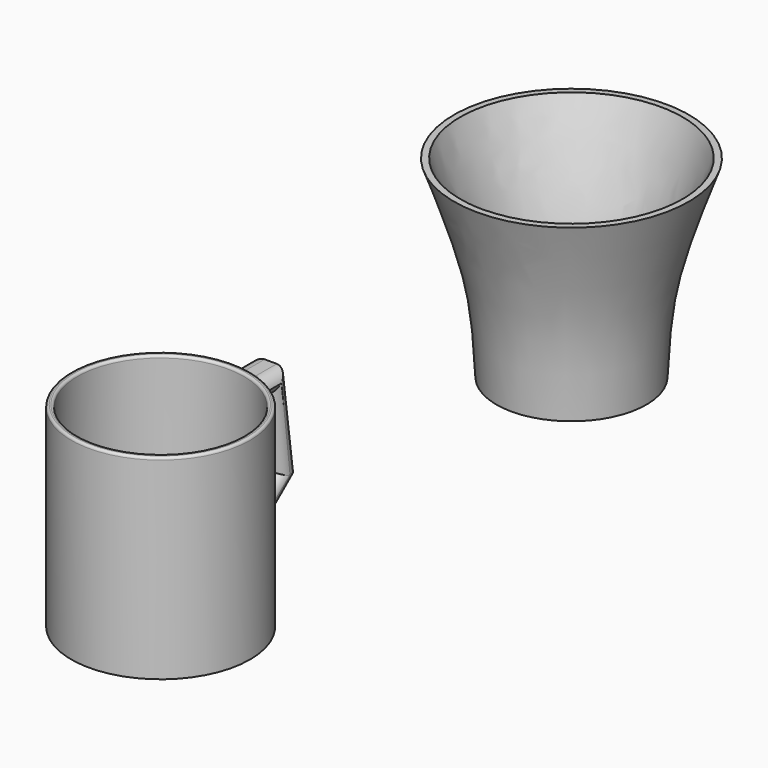
from build123d import *

# Parameters (mm, degrees)
F0_R          = 36.9971059263
F1_DEPTH      = 80.772
F2_T          = -2.54
F3_R          = 1
F5_DEPTH      = 7.5
F6_T1_DEPTH   = 65.9582815791
F6_T6_DEPTH   = 45.598795265
F6_S7_R       = 36.9971059263
F6_T8_DEPTH   = 25
F6_T12_DEPTH  = 57.9884008933
F6_S13_R      = 36.9971059263
F6_T14_DEPTH  = 33
F6_T18_DEPTH  = 44.3714568285
F6_S19_R      = 36.9971059263
F6_T20_DEPTH  = 26
F6_T25_DEPTH  = 54.3686230344
F6_T31_DEPTH  = 38.2201202214
F6_S32_R      = 36.9971059263
F6_T33_DEPTH  = 21
F6_T38_DEPTH  = 45.598795265
F6_S39_R      = 36.9971059263
F6_T40_DEPTH  = 25
F6_T44_DEPTH  = 38.2201202214
F6_S45_R      = 36.9971059263
F6_T46_DEPTH  = 21
F6_T51_DEPTH  = 54.3686230344
F6_T57_DEPTH  = 44.3714568285
F6_S58_R      = 36.9971059263
F6_T59_DEPTH  = 26
F6_T64_DEPTH  = 57.9884008933
F6_S65_R      = 36.9971059263
F6_T66_DEPTH  = 33
F6_T71_DEPTH  = 44.3714568285
F6_T76_DEPTH  = 54.3686230344
F6_T84_DEPTH  = 25.7201202214
F6_T89_DEPTH  = 54.3686230344
F6_T97_DEPTH  = 25.7201202214
F6_T102_DEPTH = 54.3686230344
F6_T110_DEPTH = 44.3714568285
F6_T115_DEPTH = 54.3686230344
F9_T          = -2.5


# Not quite as in the source:
# - a fillet or chamfer that OpenCascade refuses, or shapes differently, is made with other operations: its cross-section is extruded or revolved along the edge and cut away or added


with BuildPart() as f1:
    # F0 (on Top) → F1 (new body)
    with BuildSketch(Plane.XY):
        Circle(F0_R)
    extrude(amount=F1_DEPTH)

    # F2
    f2_openings = [f1.faces().sort_by_distance(p)[0] for p in [
        (0, 0, 80.772),
    ]]
    offset(amount=F2_T, openings=f2_openings)

    # F3
    f3_edges = [f1.edges().sort_by_distance(p)[0] for p in [
        (-34.457106, 0, 80.772),
        (-36.997106, 0, 80.772),
    ]]
    fillet(f3_edges, radius=F3_R)

    # F4 (on Right) → F5 (join, symmetric)
    with BuildSketch(Plane.YZ):
        Polygon((56.8772740662, 73.2908397913), (36.2784788013, 73.2908397913), (36.2784788013, 65.2972832322), (49.4985990226, 65.2972832322), (52.5730475783, 36.0900275409), (36.8933677673, 24.7145723552), (36.8933677673, 11.8018947542), (62.411274761, 32.7081382275), align=None)
    extrude(amount=F5_DEPTH, both=True)

    # F6: fillet of radius 5 on 12 edges, made by hand

    # F6_s2 → F6_t1 (cut)
    with BuildSketch(Plane(origin=(0, -1.5505079286, 11.3703998263), x_dir=(1, 0, 0), z_dir=(0, -0.1351131073, 0.9908301813))):
        with BuildLine():
            ThreePointArc((7.5, 61.2582728789), (6.0355339059, 64.7938067849), (2.5, 66.2582728789))
            Line((2.5, 66.2582728789), (7.5, 66.2582728789))
            Line((7.5, 66.2582728789), (7.5, 61.2582728789))
        make_face()
        with BuildLine():
            ThreePointArc((-7.5, 61.2582728789), (-6.0355339059, 64.7938067849), (-2.5, 66.2582728789))
            Line((-2.5, 66.2582728789), (-7.5, 66.2582728789))
            Line((-7.5, 66.2582728789), (-7.5, 61.2582728789))
        make_face()
    extrude(amount=F6_T1_DEPTH, mode=Mode.SUBTRACT)


with BuildPart() as f6_tool4:
    # F6_s5 → F6_t6 (new body)
    with BuildSketch(Plane.XZ.offset(-69.3772740662)):
        with BuildLine():
            ThreePointArc((2.5, 73.2908397913), (6.0355339059, 71.8263736972), (7.5, 68.2908397913))
            Line((7.5, 68.2908397913), (7.5, 73.2908397913))
            Line((7.5, 73.2908397913), (2.5, 73.2908397913))
        make_face()
    extrude(amount=F6_T6_DEPTH)

    # F6_s7 → F6_t8 (cut, symmetric)
    with BuildSketch(Plane.XY.offset(70.8)):
        Circle(F6_S7_R)
    extrude(amount=F6_T8_DEPTH, both=True, mode=Mode.SUBTRACT)


with BuildPart() as f1_1:
    add(f1.part)

    # F6_t3: cut F6_tool4
    add(f6_tool4.part, mode=Mode.SUBTRACT)


with BuildPart() as f6_tool10:
    # F6_s11 → F6_t12 (new body)
    with BuildSketch(Plane(origin=(0, 18.192122961, 14.9043944715), x_dir=(1, 0, 0), z_dir=(0, 0.7735417996, 0.6337452834))):
        with BuildLine():
            ThreePointArc((2.5, 14.2517389045), (6.0355339059, 12.7872728104), (7.5, 9.2517389045))
            Line((7.5, 9.2517389045), (7.5, 14.2517389045))
            Line((7.5, 14.2517389045), (2.5, 14.2517389045))
        make_face()
    extrude(amount=F6_T12_DEPTH)

    # F6_s13 → F6_t14 (cut, symmetric)
    with BuildSketch(Plane.XY.offset(24.2)):
        Circle(F6_S13_R)
    extrude(amount=F6_T14_DEPTH, both=True, mode=Mode.SUBTRACT)


with BuildPart() as f1_2:
    add(f1_1.part)

    # F6_t9: cut F6_tool10
    add(f6_tool10.part, mode=Mode.SUBTRACT)


with BuildPart() as f6_tool16:
    # F6_s17 → F6_t18 (new body)
    with BuildSketch(Plane(origin=(0, 61.7158510594, 44.7742496301), x_dir=(1, 0, 0), z_dir=(0, -0.8094218184, -0.587227656))):
        with BuildLine():
            ThreePointArc((2.5, -1.6602917777), (6.0355339059, -3.1247578718), (7.5, -6.6602917777))
            Line((7.5, -6.6602917777), (7.5, -1.6602917777))
            Line((7.5, -1.6602917777), (2.5, -1.6602917777))
        make_face()
    extrude(amount=F6_T18_DEPTH)

    # F6_s19 → F6_t20 (cut, symmetric)
    with BuildSketch(Plane.XY.offset(28.4)):
        Circle(F6_S19_R)
    extrude(amount=F6_T20_DEPTH, both=True, mode=Mode.SUBTRACT)

    split(bisect_by=Plane(origin=(0, 55.754223012, 5.868866703), x_dir=(1, 0, 0), z_dir=(0, -0.9945054508, -0.1046848043)), keep=Keep.TOP)


with BuildPart() as f1_3:
    add(f1_2.part)

    # F6_t15: cut F6_tool16
    add(f6_tool16.part, mode=Mode.SUBTRACT)


with BuildPart() as f6_tool23:
    # F6_s24 → F6_t25 (new body)
    with BuildSketch(Plane(origin=(0, -7.5641840435, 71.8597346646), x_dir=(1, 0, 0), z_dir=(0, 0.1046848043, -0.9945054508))):
        with BuildLine():
            ThreePointArc((7.5, -61.062259855), (6.0355339059, -57.5267259491), (2.5, -56.062259855))
            Line((2.5, -56.062259855), (7.5, -56.062259855))
            Line((7.5, -56.062259855), (7.5, -61.062259855))
        make_face()
    extrude(amount=F6_T25_DEPTH)

    split(bisect_by=Plane.XY.offset(65.2972832322), keep=Keep.BOTTOM)

    split(bisect_by=Plane(origin=(0, 0.9749692488, -1.3438763898), x_dir=(1, 0, 0), z_dir=(0, -0.587227656, 0.8094218184)), keep=Keep.TOP)


with BuildPart() as f1_4:
    add(f1_3.part)

    # F6_t22: cut F6_tool23
    add(f6_tool23.part, mode=Mode.SUBTRACT)


with BuildPart() as f6_tool29:
    # F6_s30 → F6_t31 (new body)
    with BuildSketch(Plane.XZ.offset(-23.7784788013)):
        with BuildLine():
            ThreePointArc((2.5, 65.2972832322), (6.0355339059, 66.7617493263), (7.5, 70.2972832322))
            Line((7.5, 70.2972832322), (7.5, 65.2972832322))
            Line((7.5, 65.2972832322), (2.5, 65.2972832322))
        make_face()
    extrude(amount=-F6_T31_DEPTH)

    # F6_s32 → F6_t33 (cut, symmetric)
    with BuildSketch(Plane.XY.offset(67.8)):
        Circle(F6_S32_R)
    extrude(amount=F6_T33_DEPTH, both=True, mode=Mode.SUBTRACT)

    split(bisect_by=Plane(origin=(0, 55.754223012, 5.868866703), x_dir=(1, 0, 0), z_dir=(0, -0.9945054508, -0.1046848043)), keep=Keep.TOP)


with BuildPart() as f1_5:
    add(f1_4.part)

    # F6_t28: cut F6_tool29
    add(f6_tool29.part, mode=Mode.SUBTRACT)


with BuildPart() as f6_tool36:
    # F6_s37 → F6_t38 (new body)
    with BuildSketch(Plane.XZ.offset(-69.3772740662)):
        with BuildLine():
            ThreePointArc((-2.5, 73.2908397913), (-6.0355339059, 71.8263736972), (-7.5, 68.2908397913))
            Line((-7.5, 68.2908397913), (-7.5, 73.2908397913))
            Line((-7.5, 73.2908397913), (-2.5, 73.2908397913))
        make_face()
    extrude(amount=F6_T38_DEPTH)

    # F6_s39 → F6_t40 (cut, symmetric)
    with BuildSketch(Plane.XY.offset(70.8)):
        Circle(F6_S39_R)
    extrude(amount=F6_T40_DEPTH, both=True, mode=Mode.SUBTRACT)


with BuildPart() as f1_6:
    add(f1_5.part)

    # F6_t35: cut F6_tool36
    add(f6_tool36.part, mode=Mode.SUBTRACT)


with BuildPart() as f6_tool42:
    # F6_s43 → F6_t44 (new body)
    with BuildSketch(Plane.XZ.offset(-23.7784788013)):
        with BuildLine():
            ThreePointArc((-2.5, 65.2972832322), (-6.0355339059, 66.7617493263), (-7.5, 70.2972832322))
            Line((-7.5, 70.2972832322), (-7.5, 65.2972832322))
            Line((-7.5, 65.2972832322), (-2.5, 65.2972832322))
        make_face()
    extrude(amount=-F6_T44_DEPTH)

    # F6_s45 → F6_t46 (cut, symmetric)
    with BuildSketch(Plane.XY.offset(67.8)):
        Circle(F6_S45_R)
    extrude(amount=F6_T46_DEPTH, both=True, mode=Mode.SUBTRACT)

    split(bisect_by=Plane(origin=(0, 55.754223012, 5.868866703), x_dir=(1, 0, 0), z_dir=(0, -0.9945054508, -0.1046848043)), keep=Keep.TOP)


with BuildPart() as f1_7:
    add(f1_6.part)

    # F6_t41: cut F6_tool42
    add(f6_tool42.part, mode=Mode.SUBTRACT)


with BuildPart() as f6_tool49:
    # F6_s50 → F6_t51 (new body)
    with BuildSketch(Plane(origin=(0, -7.5641840435, 71.8597346646), x_dir=(1, 0, 0), z_dir=(0, 0.1046848043, -0.9945054508))):
        with BuildLine():
            ThreePointArc((-2.5, -56.062259855), (-6.0355339059, -57.5267259491), (-7.5, -61.062259855))
            Line((-7.5, -61.062259855), (-7.5, -56.062259855))
            Line((-7.5, -56.062259855), (-2.5, -56.062259855))
        make_face()
    extrude(amount=F6_T51_DEPTH)

    split(bisect_by=Plane.XY.offset(65.2972832322), keep=Keep.BOTTOM)

    split(bisect_by=Plane(origin=(0, 0.9749692488, -1.3438763898), x_dir=(1, 0, 0), z_dir=(0, -0.587227656, 0.8094218184)), keep=Keep.TOP)


with BuildPart() as f1_8:
    add(f1_7.part)

    # F6_t48: cut F6_tool49
    add(f6_tool49.part, mode=Mode.SUBTRACT)


with BuildPart() as f6_tool55:
    # F6_s56 → F6_t57 (new body)
    with BuildSketch(Plane(origin=(0, 61.7158510594, 44.7742496301), x_dir=(1, 0, 0), z_dir=(0, -0.8094218184, -0.587227656))):
        with BuildLine():
            ThreePointArc((-2.5, -1.6602917777), (-6.0355339059, -3.1247578718), (-7.5, -6.6602917777))
            Line((-7.5, -6.6602917777), (-7.5, -1.6602917777))
            Line((-7.5, -1.6602917777), (-2.5, -1.6602917777))
        make_face()
    extrude(amount=F6_T57_DEPTH)

    # F6_s58 → F6_t59 (cut, symmetric)
    with BuildSketch(Plane.XY.offset(28.4)):
        Circle(F6_S58_R)
    extrude(amount=F6_T59_DEPTH, both=True, mode=Mode.SUBTRACT)

    split(bisect_by=Plane(origin=(0, 55.754223012, 5.868866703), x_dir=(1, 0, 0), z_dir=(0, -0.9945054508, -0.1046848043)), keep=Keep.TOP)


with BuildPart() as f1_9:
    add(f1_8.part)

    # F6_t54: cut F6_tool55
    add(f6_tool55.part, mode=Mode.SUBTRACT)


with BuildPart() as f6_tool62:
    # F6_s63 → F6_t64 (new body)
    with BuildSketch(Plane(origin=(0, 18.192122961, 14.9043944715), x_dir=(1, 0, 0), z_dir=(0, 0.7735417996, 0.6337452834))):
        with BuildLine():
            ThreePointArc((-2.5, 14.2517389045), (-6.0355339059, 12.7872728104), (-7.5, 9.2517389045))
            Line((-7.5, 9.2517389045), (-7.5, 14.2517389045))
            Line((-7.5, 14.2517389045), (-2.5, 14.2517389045))
        make_face()
    extrude(amount=F6_T64_DEPTH)

    # F6_s65 → F6_t66 (cut, symmetric)
    with BuildSketch(Plane.XY.offset(24.2)):
        Circle(F6_S65_R)
    extrude(amount=F6_T66_DEPTH, both=True, mode=Mode.SUBTRACT)


with BuildPart() as f1_10:
    add(f1_9.part)

    # F6_t61: cut F6_tool62
    add(f6_tool62.part, mode=Mode.SUBTRACT)


with BuildPart() as f6_tool69:
    # F6_s70 → F6_t71 (new body)
    with BuildSketch(Plane(origin=(0, 61.7158510594, 44.7742496301), x_dir=(1, 0, 0), z_dir=(0, -0.8094218184, -0.587227656))):
        with BuildLine():
            ThreePointArc((2.5, -1.6602917777), (6.0355339059, -3.1247578718), (7.5, -6.6602917777))
            Line((7.5, -6.6602917777), (7.5, -1.6602917777))
            Line((7.5, -1.6602917777), (2.5, -1.6602917777))
        make_face()
    extrude(amount=F6_T71_DEPTH)

    split(bisect_by=Plane(origin=(0, 55.754223012, 5.868866703), x_dir=(1, 0, 0), z_dir=(0, 0.9945054508, 0.1046848043)), keep=Keep.TOP)

    split(bisect_by=Plane(origin=(0, 65.6506965311, 8.9523611345), x_dir=(1, 0, 0), z_dir=(0, -0.9908301813, -0.1351131073)), keep=Keep.TOP)


with BuildPart() as f6_tool74:
    # F6_s75 → F6_t76 (new body)
    with BuildSketch(Plane(origin=(0, -7.5641840435, 71.8597346646), x_dir=(1, 0, 0), z_dir=(0, 0.1046848043, -0.9945054508))):
        with BuildLine():
            ThreePointArc((7.5, -61.062259855), (6.0355339059, -57.5267259491), (2.5, -56.062259855))
            Line((2.5, -56.062259855), (7.5, -56.062259855))
            Line((7.5, -56.062259855), (7.5, -61.062259855))
        make_face()
    extrude(amount=F6_T76_DEPTH)

    split(bisect_by=Plane(origin=(0, 9.0319723111, -11.0243157599), x_dir=(1, 0, 0), z_dir=(0, -0.6337452834, 0.7735417996)), keep=Keep.TOP)

    split(bisect_by=Plane(origin=(0, 0.9749692488, -1.3438763898), x_dir=(1, 0, 0), z_dir=(0, 0.587227656, -0.8094218184)), keep=Keep.TOP)


with BuildPart() as f6_tool69_1:
    add(f6_tool69.part)

    # F6_t79: intersect F6_tool74
    add(f6_tool74.part, mode=Mode.INTERSECT)


with BuildPart() as f1_11:
    add(f1_10.part)

    # F6_t67: cut F6_tool69
    add(f6_tool69_1.part, mode=Mode.SUBTRACT)


with BuildPart() as f6_tool82:
    # F6_s83 → F6_t84 (new body)
    with BuildSketch(Plane.XZ.offset(-36.2784788013)):
        with BuildLine():
            ThreePointArc((2.5, 65.2972832322), (6.0355339059, 66.7617493263), (7.5, 70.2972832322))
            Line((7.5, 70.2972832322), (7.5, 65.2972832322))
            Line((7.5, 65.2972832322), (2.5, 65.2972832322))
        make_face()
    extrude(amount=-F6_T84_DEPTH)

    split(bisect_by=Plane(origin=(0, 55.754223012, 5.868866703), x_dir=(1, 0, 0), z_dir=(0, 0.9945054508, 0.1046848043)), keep=Keep.TOP)

    split(bisect_by=Plane(origin=(0, 65.6506965311, 8.9523611345), x_dir=(1, 0, 0), z_dir=(0, -0.9908301813, -0.1351131073)), keep=Keep.TOP)


with BuildPart() as f6_tool87:
    # F6_s88 → F6_t89 (new body)
    with BuildSketch(Plane(origin=(0, -7.5641840435, 71.8597346646), x_dir=(1, 0, 0), z_dir=(0, 0.1046848043, -0.9945054508))):
        with BuildLine():
            ThreePointArc((7.5, -61.062259855), (6.0355339059, -57.5267259491), (2.5, -56.062259855))
            Line((2.5, -56.062259855), (7.5, -56.062259855))
            Line((7.5, -56.062259855), (7.5, -61.062259855))
        make_face()
    extrude(amount=F6_T89_DEPTH)

    split(bisect_by=Plane.XY.offset(65.2972832322), keep=Keep.TOP)

    split(bisect_by=Plane.XY.offset(73.2908397913), keep=Keep.BOTTOM)


with BuildPart() as f6_tool82_1:
    add(f6_tool82.part)

    # F6_t92: intersect F6_tool87
    add(f6_tool87.part, mode=Mode.INTERSECT)


with BuildPart() as f1_12:
    add(f1_11.part)

    # F6_t80: cut F6_tool82
    add(f6_tool82_1.part, mode=Mode.SUBTRACT)


with BuildPart() as f6_tool95:
    # F6_s96 → F6_t97 (new body)
    with BuildSketch(Plane.XZ.offset(-36.2784788013)):
        with BuildLine():
            ThreePointArc((-2.5, 65.2972832322), (-6.0355339059, 66.7617493263), (-7.5, 70.2972832322))
            Line((-7.5, 70.2972832322), (-7.5, 65.2972832322))
            Line((-7.5, 65.2972832322), (-2.5, 65.2972832322))
        make_face()
    extrude(amount=-F6_T97_DEPTH)

    split(bisect_by=Plane(origin=(0, 55.754223012, 5.868866703), x_dir=(1, 0, 0), z_dir=(0, 0.9945054508, 0.1046848043)), keep=Keep.TOP)

    split(bisect_by=Plane(origin=(0, 65.6506965311, 8.9523611345), x_dir=(1, 0, 0), z_dir=(0, -0.9908301813, -0.1351131073)), keep=Keep.TOP)


with BuildPart() as f6_tool100:
    # F6_s101 → F6_t102 (new body)
    with BuildSketch(Plane(origin=(0, -7.5641840435, 71.8597346646), x_dir=(1, 0, 0), z_dir=(0, 0.1046848043, -0.9945054508))):
        with BuildLine():
            ThreePointArc((-2.5, -56.062259855), (-6.0355339059, -57.5267259491), (-7.5, -61.062259855))
            Line((-7.5, -61.062259855), (-7.5, -56.062259855))
            Line((-7.5, -56.062259855), (-2.5, -56.062259855))
        make_face()
    extrude(amount=F6_T102_DEPTH)

    split(bisect_by=Plane.XY.offset(65.2972832322), keep=Keep.TOP)

    split(bisect_by=Plane.XY.offset(73.2908397913), keep=Keep.BOTTOM)


with BuildPart() as f6_tool95_1:
    add(f6_tool95.part)

    # F6_t105: intersect F6_tool100
    add(f6_tool100.part, mode=Mode.INTERSECT)


with BuildPart() as f1_13:
    add(f1_12.part)

    # F6_t93: cut F6_tool95
    add(f6_tool95_1.part, mode=Mode.SUBTRACT)


with BuildPart() as f6_tool108:
    # F6_s109 → F6_t110 (new body)
    with BuildSketch(Plane(origin=(0, 61.7158510594, 44.7742496301), x_dir=(1, 0, 0), z_dir=(0, -0.8094218184, -0.587227656))):
        with BuildLine():
            ThreePointArc((-2.5, -1.6602917777), (-6.0355339059, -3.1247578718), (-7.5, -6.6602917777))
            Line((-7.5, -6.6602917777), (-7.5, -1.6602917777))
            Line((-7.5, -1.6602917777), (-2.5, -1.6602917777))
        make_face()
    extrude(amount=F6_T110_DEPTH)

    split(bisect_by=Plane(origin=(0, 55.754223012, 5.868866703), x_dir=(1, 0, 0), z_dir=(0, 0.9945054508, 0.1046848043)), keep=Keep.TOP)

    split(bisect_by=Plane(origin=(0, 65.6506965311, 8.9523611345), x_dir=(1, 0, 0), z_dir=(0, -0.9908301813, -0.1351131073)), keep=Keep.TOP)


with BuildPart() as f6_tool113:
    # F6_s114 → F6_t115 (new body)
    with BuildSketch(Plane(origin=(0, -7.5641840435, 71.8597346646), x_dir=(1, 0, 0), z_dir=(0, 0.1046848043, -0.9945054508))):
        with BuildLine():
            ThreePointArc((-2.5, -56.062259855), (-6.0355339059, -57.5267259491), (-7.5, -61.062259855))
            Line((-7.5, -61.062259855), (-7.5, -56.062259855))
            Line((-7.5, -56.062259855), (-2.5, -56.062259855))
        make_face()
    extrude(amount=F6_T115_DEPTH)

    split(bisect_by=Plane(origin=(0, 9.0319723111, -11.0243157599), x_dir=(1, 0, 0), z_dir=(0, -0.6337452834, 0.7735417996)), keep=Keep.TOP)

    split(bisect_by=Plane(origin=(0, 0.9749692488, -1.3438763898), x_dir=(1, 0, 0), z_dir=(0, 0.587227656, -0.8094218184)), keep=Keep.TOP)


with BuildPart() as f6_tool108_1:
    add(f6_tool108.part)

    # F6_t118: intersect F6_tool113
    add(f6_tool113.part, mode=Mode.INTERSECT)


with BuildPart() as f1_14:
    add(f1_13.part)

    # F6_t106: cut F6_tool108
    add(f6_tool108_1.part, mode=Mode.SUBTRACT)


with BuildPart() as f8:
    # F7 (on Right) → F8 (revolve)
    with BuildSketch(Plane.YZ):
        with BuildLine():
            Line((212.3078554869, 4.5110611245), (212.3078554869, 85.1721689105))
            Line((212.3078554869, 85.1721689105), (163.7043654919, 84.1380506754))
            add(Edge.make_bspline(
                [(181.284353137, 4.5110611245), (180.7402742969, 15.9545446682), (179.5714275307, 40.538626511), (169.2313225835, 68.9511089476), (163.7043654919, 84.1380506754)],
                knots=[0, 0, 0, 0, 0.4654834627, 1, 1, 1, 1], degree=3))
            Line((181.284353137, 4.5110611245), (212.3078554869, 4.5110611245))
        make_face()
    revolve(axis=Axis((0, 212.3078554869, 44.8416150175), (0, 0, -1)))

    # F9
    f9_openings = [f8.faces().sort_by_distance(p)[0] for p in [
        (0, 236.6096, 84.65511),
    ]]
    offset(amount=F9_T, openings=f9_openings)


solid = Compound([f1_14.part, f8.part])
